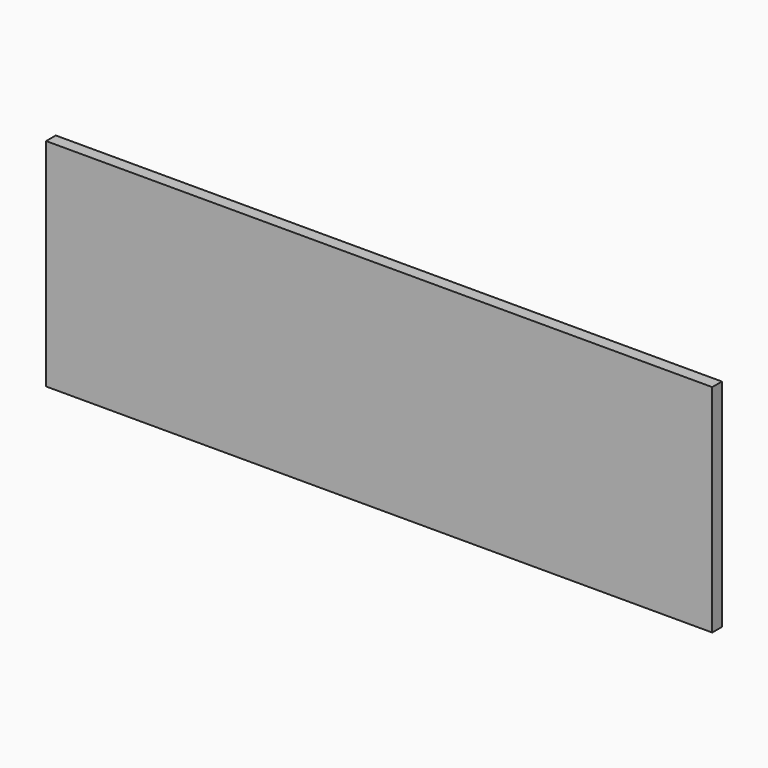
from build123d import *

# Parameters (mm, degrees)
F0_W     = 110
F0_H     = 35.6789995135
F1_DEPTH = 2


with BuildPart() as f1:
    # F0 (on Front) → F1 (new body)
    with BuildSketch(Plane.XZ):
        Rectangle(F0_W, F0_H)
    extrude(amount=F1_DEPTH)


solid = f1.part
